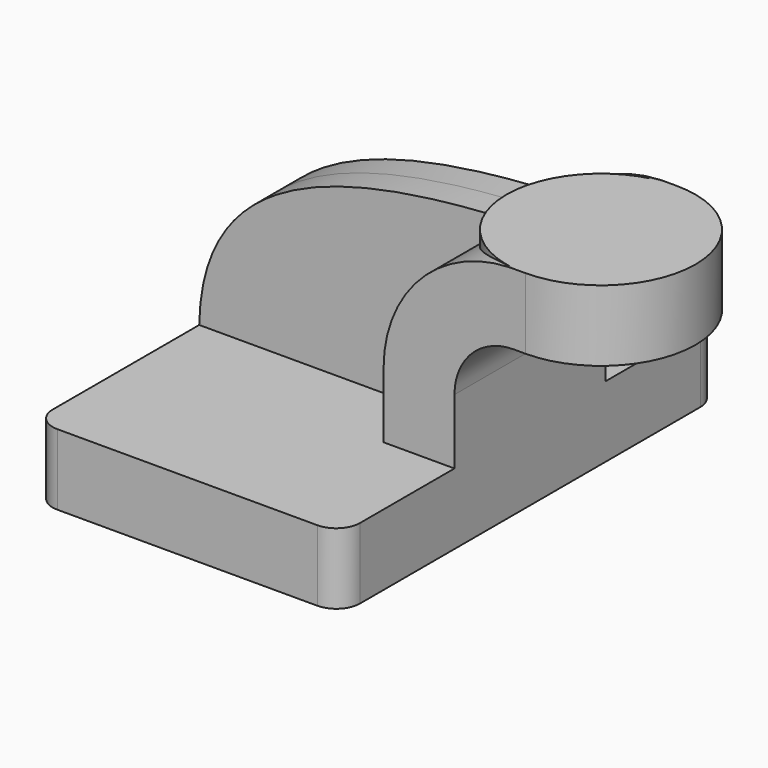
from build123d import *

# Parameters (mm, degrees)
F1_DEPTH = 63.5
F2_DEPTH = 25.4
F3_DEPTH = 7.9375
F5_R     = 6.35


with BuildPart() as f1:
    # F0 (on Front) → F1 (new body, symmetric)
    with BuildSketch(Plane.XZ):
        Polygon((-41.275, -9.525), (41.275, -9.525), (41.275, 9.525), (22.225, 9.525), (-41.275, 9.525), align=None)
    extrude(amount=F1_DEPTH, both=True)

    # F0 (on Front) → F2 (join, symmetric)
    with BuildSketch(Plane.XZ):
        with BuildLine():
            Line((22.225, 9.525), (41.275, 9.525))
            Line((41.275, 9.525), (41.275, 27.0002))
            ThreePointArc((41.275, 27.0002), (45.9246798487, 38.2255201513), (57.15, 42.8752))
            Line((57.15, 42.8752), (60.325, 42.8752))
            Line((60.325, 42.8752), (60.325, 61.9252))
            Line((60.325, 61.9252), (57.15, 61.9252))
            add(Edge.make_bspline(
                [(55.950364042, 61.9045908208), (56.3494203194, 61.9119140361), (56.7493016333, 61.9187812014), (57.15, 61.9252)],
                knots=[110.7227393915, 110.7227393915, 110.7227393915, 110.7227393915, 111.5045361635, 111.5045361635, 111.5045361635, 111.5045361635], degree=3))
            ThreePointArc((55.950364042, 61.9045908208), (32.0337412138, 51.2680628969), (22.225, 27.0002))
            Line((22.225, 27.0002), (22.225, 9.525))
        make_face()
    extrude(amount=F2_DEPTH, both=True)

    # F0 (on Front) → F3 (join, symmetric)
    with BuildSketch(Plane.XZ):
        with BuildLine():
            add(Edge.make_bspline(
                [(-41.275, 9.525), (-40.5345981749, 50.6828617224), (-0.5663750684, 60.8674332248), (55.950364042, 61.9045908208)],
                knots=[0, 0, 0, 0, 110.7227393915, 110.7227393915, 110.7227393915, 110.7227393915], degree=3))
            Line((-41.275, 9.525), (22.225, 9.525))
            Line((22.225, 9.525), (22.225, 27.0002))
            ThreePointArc((22.225, 27.0002), (32.0337412138, 51.2680628969), (55.950364042, 61.9045908208))
        make_face()
    extrude(amount=F3_DEPTH, both=True)

    # F0 (on Front) → F4 (revolve)
    with BuildSketch(Plane.XZ):
        Polygon((60.325, 61.9252), (60.325, 42.8752), (85.725, 42.8752), (85.725, 47.9196608067), (85.725, 61.9252), align=None)
    revolve(axis=Axis((60.325, 0, 52.3875), (0, 0, 1)))

    # F5
    f5_edges = [f1.edges().sort_by_distance(p)[0] for p in [
        (41.275, -63.5, 0),
        (-41.275, -63.5, 0),
        (41.275, 63.5, 0),
        (-41.275, 63.5, 0),
    ]]
    fillet(f5_edges, radius=F5_R)


solid = f1.part
